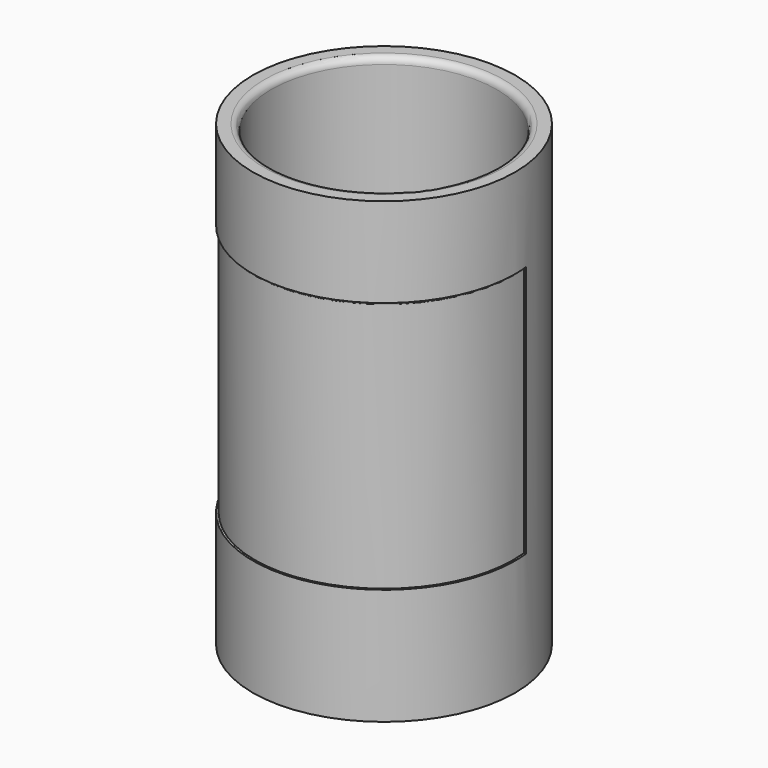
from build123d import *

# Parameters (mm, degrees)
F0_R     = 39.5
F1_DEPTH = 138
F2_W     = 34
F2_H     = 130
F6_DEPTH = 38
F7_R     = 0.59999
F8_R     = 2


# Not quite as in the source:
# - a fillet or chamfer is up to 0.001 mm smaller than in the source, because OpenCascade refuses the exact size


with BuildPart() as f1:
    # F0 (on Top) → F1 (new body)
    with BuildSketch(Plane.XY):
        Circle(F0_R)
    extrude(amount=F1_DEPTH)

    # F2 (on Front) → F3 (revolve, cut)
    with BuildSketch(Plane.XZ):
        with Locations((-17, 73)):
            Rectangle(F2_W, F2_H)
    revolve(axis=Axis((0, 0, 73), (0, 0, 1)), mode=Mode.SUBTRACT)

    # F5 (on plane+point) → F6 (cut, symmetric)
    with BuildSketch(Plane.XY.offset(73)):
        with BuildLine():
            Line((-38.6499451858, 4.4036050156), (-39.2460882992, 4.4715269438))
            ThreePointArc((-39.2460882992, 4.4715269438), (0, -39.5), (39.2460882992, 4.4715269438))
            Line((39.2460882992, 4.4715269438), (38.6499451858, 4.4036050156))
            ThreePointArc((38.6499451858, 4.4036050156), (0, -38.9), (-38.6499451858, 4.4036050156))
        make_face()
    extrude(amount=F6_DEPTH, both=True, mode=Mode.SUBTRACT)

    # F7 (radius 0.6 in the source; OpenCascade refuses exactly that, so slightly less here)
    f7_edges = [f1.edges().sort_by_distance(p)[0] for p in [
        (0, -38.9, 111),
    ]]
    fillet(f7_edges, radius=F7_R)

    # F8
    f8_edges = [f1.edges().sort_by_distance(p)[0] for p in [
        (34, 0, 8),
        (34, 0, 138),
    ]]
    fillet(f8_edges, radius=F8_R)


solid = f1.part
